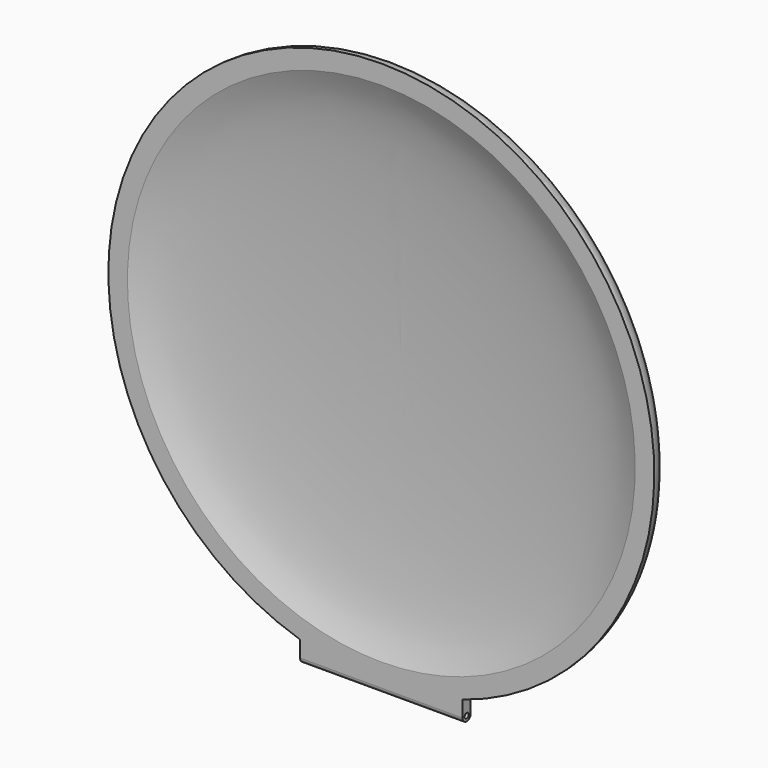
from build123d import *

# Parameters (mm, degrees)
F3_DEPTH = 1.27
F4_R     = 0.3175
F5_DEPTH = 44.2922501


# Not quite as in the source:
# - the dataset's text gives a spline's control points without its knots; the knots are read off the source's solid


with BuildPart() as f1:
    # F0 (on Right) → F1 (revolve)
    with BuildSketch(Plane.YZ):
        with BuildLine():
            Line((0, 34.13125), (0, 31.75))
            add(Edge.make_bspline(
                [(0, 31.75), (0.5742670905, 30.3542906008), (2.3414834837, 25.8865164681), (3.175, 10.5516560434), (3.175, 0)],
                knots=[0, 0, 0, 0, 0.3124675666, 1, 1, 1, 1], degree=3))
            Line((3.175, 0), (5.55625, 0))
            add(Edge.make_bspline(
                [(2.2021322713, 32.6560712016), (2.3186413793, 32.3729053021), (2.5576698716, 31.7878917938), (2.9240965193, 30.812098832), (3.2829237449, 29.7062776723), (3.6213582396, 28.4414870624), (3.9333609229, 26.9775001767), (4.2135585587, 25.2856930459), (4.4651056247, 23.3880591837), (4.7658122637, 20.5979082433), (5.0781689931, 16.6702210435), (5.3509257758, 11.4172981506), (5.5180630854, 5.8010058197), (5.55625, 1.9340677683), (5.55625, 0)],
                knots=[1e-10, 1e-10, 1e-10, 1e-10, 0.0625000001, 0.1250000001, 0.1875000001, 0.2500000001, 0.3125000001, 0.3750000001, 0.4375000001, 0.5, 0.625, 0.75, 0.875, 1, 1, 1, 1], degree=3))
            ThreePointArc((2.2021322713, 32.6560712016), (1.3252866697, 33.728374789), (0, 34.13125))
        make_face()
    revolve(axis=Axis((0, 4.365625, 0), (0, -1, 0)))

    # F2 (on face) → F3 (join)
    with BuildSketch(Plane.XZ):
        with BuildLine():
            Line((-10.16, -30.0805069771), (-10.16, -35.2621069771))
            Line((-10.16, -35.2621069771), (10.16, -35.2621069771))
            Line((10.16, -35.2621069771), (10.16, -30.0805069771))
            ThreePointArc((10.16, -30.0805069771), (0, -31.75), (-10.16, -30.0805069771))
        make_face()
    extrude(amount=-F3_DEPTH)

    # F4 (on face) → F5 (cut, through all)
    with BuildSketch(Plane.YZ.offset(10.16)):
        with Locations((0.635, -34.6159934103)):
            Circle(F4_R)
        with BuildLine():
            Line((1.27, -35.2621069771), (1.27, -34.6159934103))
            ThreePointArc((1.27, -34.6159934103), (0.635, -35.2509934103), (0, -34.6159934103))
            Line((0, -34.6159934103), (0, -35.2621069771))
            Line((0, -35.2621069771), (1.27, -35.2621069771))
        make_face()
    extrude(amount=-F5_DEPTH, mode=Mode.SUBTRACT)


solid = f1.part
